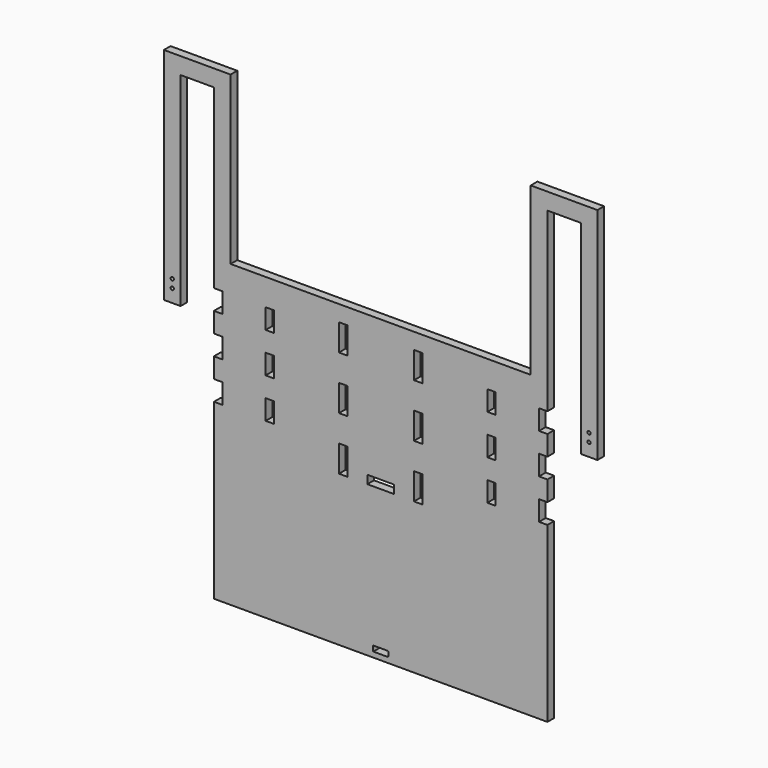
from build123d import *

# Parameters (mm, degrees)
F0_W     = 12.7
F0_H     = 6.35
F0_W_2   = 6.35
F0_H_2   = 77.47
F0_R     = 0.635
F0_W_3   = 3.175
F0_H_3   = 7.62
F0_H_4   = 10.16
F0_W_4   = 10.16
F0_H_5   = 3.175
F1_DEPTH = 3.175


# Not quite as in the source:
# - a feature names something its author has since deleted; it is built from what else it names


with BuildPart() as f1:
    # F0 (on Front) → F1 (new body)
    with BuildSketch(Plane.XZ):
        Polygon((-63.5, 57.15), (-57.15, 57.15), (-57.15, 120.65), (-63.5, 120.65), (-63.5, 114.3), align=None)
        with Locations((-69.85, 117.475)):
            Rectangle(F0_W, F0_H)
        with Locations((-79.375, 117.475)):
            Rectangle(F0_W_2, F0_H)
        with Locations((-79.375, 75.565)):
            Rectangle(F0_W_2, F0_H_2)
        with Locations((-79.375, 41.7701676488)):
            Circle(F0_R, mode=Mode.SUBTRACT)
        with Locations((-79.375, 44.9451676488)):
            Circle(F0_R, mode=Mode.SUBTRACT)
        Polygon((57.15, 57.15), (63.5, 57.15), (63.5, 114.3), (63.5, 120.65), (57.15, 120.65), align=None)
        Polygon((63.5, 120.65), (63.5, 114.3), (76.2, 114.3), (82.55, 114.3), (82.55, 120.65), align=None)
        with Locations((79.375, 75.565)):
            Rectangle(F0_W_2, F0_H_2)
        with Locations((79.375, 41.7701676488)):
            Circle(F0_R, mode=Mode.SUBTRACT)
        with Locations((79.375, 44.9451676488)):
            Circle(F0_R, mode=Mode.SUBTRACT)
        Polygon((63.5, 46.99), (63.5, 57.15), (57.15, 57.15), (-57.15, 57.15), (-63.5, 57.15), (-63.5, 46.99), (-60.325, 46.99), (-60.325, 39.37), (-63.5, 39.37), (-63.5, 31.75), (-60.325, 31.75), (-60.325, 24.13), (-63.5, 24.13), (-63.5, 16.51), (-60.325, 16.51), (-60.325, 8.89), (-63.5, 8.89), (-63.5, -57.15), (63.5, -57.15), (63.5, 8.89), (60.325, 8.89), (60.325, 16.51), (63.5, 16.51), (63.5, 24.13), (60.325, 24.13), (60.325, 31.75), (63.5, 31.75), (63.5, 39.37), (60.325, 39.37), (60.325, 46.99), align=None)
        with Locations((-42.2275, 12.7)):
            Rectangle(F0_W_3, F0_H_3, mode=Mode.SUBTRACT)
        with Locations((-42.2275, 27.94)):
            Rectangle(F0_W_3, F0_H_3, mode=Mode.SUBTRACT)
        with Locations((-14.2875, 5.3341257808)):
            Rectangle(F0_W_3, F0_H_4, mode=Mode.SUBTRACT)
        with Locations((-14.2875, 25.6541257808)):
            Rectangle(F0_W_3, F0_H_4, mode=Mode.SUBTRACT)
        with BuildLine():
            ThreePointArc((2.8175964356, -53.0858742192), (2.9972, -54.1078126547), (2.8175964356, -55.1297510902))
            Line((2.8175964356, -55.1297510902), (-2.8175964356, -55.1297510902))
            ThreePointArc((-2.8175964356, -55.1297510902), (-2.9972, -54.1078126547), (-2.8175964356, -53.0858742192))
            Line((-2.8175964356, -53.0858742192), (2.8175964356, -53.0858742192))
        make_face(mode=Mode.SUBTRACT)
        with Locations((0, 1.8416257808)):
            Rectangle(F0_W_4, F0_H_5, mode=Mode.SUBTRACT)
        with Locations((14.2875, 5.3341257808)):
            Rectangle(F0_W_3, F0_H_4, mode=Mode.SUBTRACT)
        with Locations((14.2875, 25.6541257808)):
            Rectangle(F0_W_3, F0_H_4, mode=Mode.SUBTRACT)
        with Locations((42.2275, 12.7)):
            Rectangle(F0_W_3, F0_H_3, mode=Mode.SUBTRACT)
        with Locations((42.2275, 27.94)):
            Rectangle(F0_W_3, F0_H_3, mode=Mode.SUBTRACT)
        with Locations((-42.2275, 43.18)):
            Rectangle(F0_W_3, F0_H_3, mode=Mode.SUBTRACT)
        with Locations((-14.2875, 45.9741257808)):
            Rectangle(F0_W_3, F0_H_4, mode=Mode.SUBTRACT)
        with Locations((14.2875, 45.9741257808)):
            Rectangle(F0_W_3, F0_H_4, mode=Mode.SUBTRACT)
        with Locations((42.2275, 43.18)):
            Rectangle(F0_W_3, F0_H_3, mode=Mode.SUBTRACT)
    extrude(amount=F1_DEPTH)


solid = f1.part
